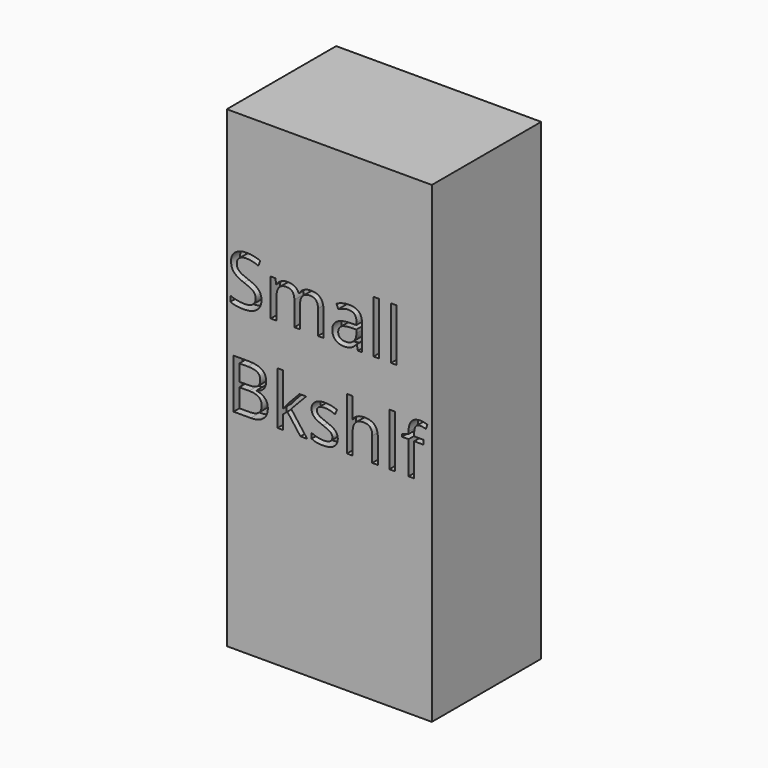
from build123d import *

# Parameters (mm, degrees)
F0_W         = 457.2
F0_H         = 1054.1
F1_DEPTH     = 152.4
F2_TEXT_SIZE = 154.288426048
F3_DEPTH     = 25.4


# Not quite as in the source:
# - Text() gives the source's letters only with a copy of the font that has no kerning and outlines rounded to 1/6400 em; it was checked with that copy


with BuildPart() as f1:
    # F0 (on Front) → F1 (new body, symmetric)
    with BuildSketch(Plane.XZ):
        Rectangle(F0_W, F0_H)
    extrude(amount=F1_DEPTH, both=True)

    # F2 (on face) → F3 (cut)
    with BuildSketch(Plane.XZ.offset(152.4)):
        with Locations((-228.6, 147.9849213346)):
            Text('Small', F2_TEXT_SIZE, font='Open Sans', text_align=(TextAlign.LEFT, TextAlign.BOTTOM))
        with Locations((-228.6, -61.8473380906)):
            Text('Bkshlf', F2_TEXT_SIZE, font='Open Sans', text_align=(TextAlign.LEFT, TextAlign.BOTTOM))
    extrude(amount=-F3_DEPTH, mode=Mode.SUBTRACT)


solid = f1.part
